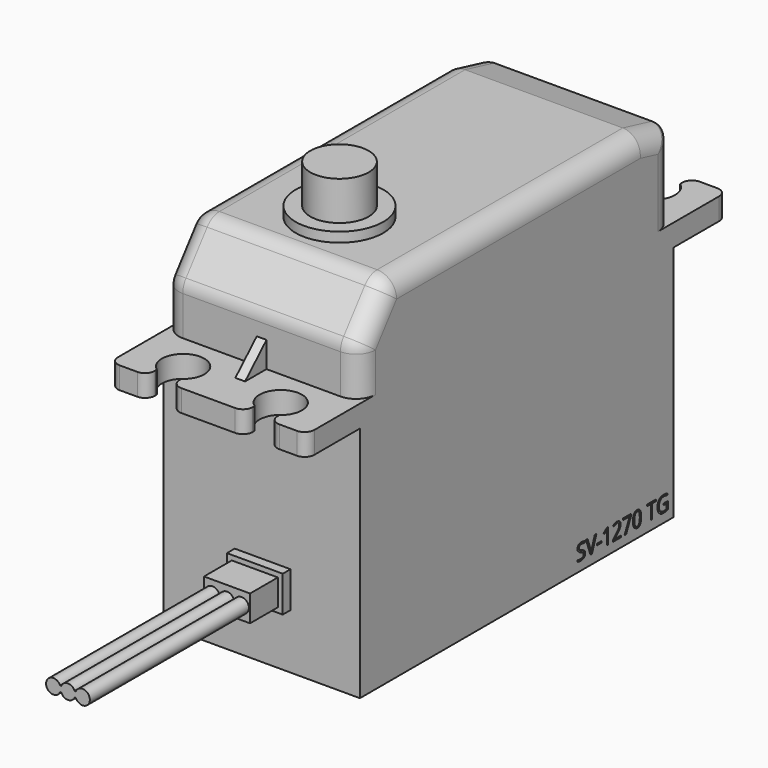
from build123d import *

# Parameters (mm, degrees)
F0_W          = 40.3
F0_H          = 24.4
F1_DEPTH      = 10.1
F2_DEPTH      = 0.5
F3_W          = 20.2
F3_H          = 27.65
F3_R          = 4.5
F3_H_2        = 5
F3_H_3        = 3
F4_DEPTH      = 1
F3_R_2        = 3
F5_DEPTH      = 4
F7_DEPTH      = 25
F8_R          = 2
F9_W          = 5.7326205064
F9_H          = 3.7
F9_W_2        = 4.7326205064
F9_H_2        = 2.7
F10_DEPTH     = 1
F11_DEPTH     = 4.57
F12_DEPTH     = 25
F13_TEXT_SIZE = 2.2495992416
F14_DEPTH     = 0.1
F15_R         = 0.5


# Not quite as in the source:
# - Text() gives the source's letters only with a copy of the font that has no kerning and outlines rounded to 1/6400 em; it was checked with that copy


with BuildPart() as f1:
    # F0 (on Right) → F1 (new body, symmetric)
    with BuildSketch(Plane.YZ):
        with Locations((0, -6.4)):
            Rectangle(F0_W, F0_H)
        Polygon((20.15, 8.05), (-20.15, 8.05), (-22.9002591223, 8.05), (-27, 8.05), (-27, 5.8), (-20.15, 5.8), (20.15, 5.8), (27.0000007004, 5.8), (27.0000007004, 8.05), (22.9000007004, 8.05), align=None)
        Polygon((12, 18.6), (-15.65, 18.6), (-20.15, 12.7771655098), (-20.15, 10.6946583837), (-20.15, 8.05), (20.15, 8.05), (20.15, 10.6946583837), (20.15, 16.6118297357), align=None)
    extrude(amount=F1_DEPTH, both=True)

    # F0 (on Right) → F2 (join, symmetric)
    with BuildSketch(Plane.YZ):
        Polygon((-20.15, 8.05), (-20.15, 10.6946583837), (-22.9002591223, 8.05), align=None)
        Polygon((22.9000007004, 8.05), (20.15, 10.6946583837), (20.15, 8.05), align=None)
    extrude(amount=F2_DEPTH, both=True)

    # F3 (on face) → F4 (cut)
    with BuildSketch(Plane.XY.offset(18.6)):
        with Locations((0, -1.825)):
            Rectangle(F3_W, F3_H)
        with Locations((0, -10.15)):
            Circle(F3_R, mode=Mode.SUBTRACT)
        with Locations((0, 14.5)):
            Rectangle(F3_W, F3_H_2)
        with Locations((0, -17.15)):
            Rectangle(F3_W, F3_H_3)
    extrude(amount=-F4_DEPTH, mode=Mode.SUBTRACT)

    # F3 (on face) → F5 (join)
    with BuildSketch(Plane.XY.offset(18.6)):
        with Locations((0, -10.15)):
            Circle(F3_R_2)
    extrude(amount=F5_DEPTH)

    # F6 (on Top) → F7 (cut)
    with BuildSketch(Plane.XY):
        with BuildLine():
            Line((0, -27), (0, -27.5084525347))
            Line((0, -27.5084525347), (10.378325358, -27.5084525347))
            Line((10.378325358, -27.5084525347), (10.378325358, -26))
            Line((10.378325358, -26), (10.1, -26))
            ThreePointArc((10.1, -26), (9.8071067812, -26.7071067812), (9.1, -27))
            Line((9.1, -27), (7.3, -27))
            ThreePointArc((7.3, -27), (6.5928932188, -26.7071067812), (6.3, -26))
            Line((6.3, -26), (6.3, -25.7791513451))
            ThreePointArc((6.3, -25.7791513451), (6.310365142, -25.734816345), (6.3393118446, -25.6996721164))
            ThreePointArc((6.3393118446, -25.6996721164), (4.9961864321, -21.7871178127), (3.7255205843, -25.7238011065))
            ThreePointArc((3.7255205843, -25.7238011065), (3.7555318396, -25.7592266373), (3.766310058, -25.8043871697))
            Line((3.766310058, -25.8043871697), (3.766310058, -26))
            ThreePointArc((3.766310058, -26), (3.4734168392, -26.7071067812), (2.766310058, -27))
            Line((2.766310058, -27), (0, -27))
        make_face()
        with BuildLine():
            Line((-10.378325358, -27.5084525347), (0, -27.5084525347))
            Line((0, -27.5084525347), (0, -27))
            Line((0, -27), (-2.766310058, -27))
            ThreePointArc((-2.766310058, -27), (-3.4734168392, -26.7071067812), (-3.766310058, -26))
            Line((-3.766310058, -26), (-3.766310058, -25.8043871697))
            ThreePointArc((-3.766310058, -25.8043871697), (-3.7555318396, -25.7592266373), (-3.7255205843, -25.7238011065))
            ThreePointArc((-3.7255205843, -25.7238011065), (-4.9961864321, -21.7871178127), (-6.3393118446, -25.6996721164))
            ThreePointArc((-6.3393118446, -25.6996721164), (-6.310365142, -25.734816345), (-6.3, -25.7791513451))
            Line((-6.3, -25.7791513451), (-6.3, -26))
            ThreePointArc((-6.3, -26), (-6.5928932188, -26.7071067812), (-7.3, -27))
            Line((-7.3, -27), (-9.1, -27))
            ThreePointArc((-9.1, -27), (-9.8071067812, -26.7071067812), (-10.1, -26))
            Line((-10.1, -26), (-10.378325358, -26))
            Line((-10.378325358, -26), (-10.378325358, -27.5084525347))
        make_face()
        with BuildLine():
            Line((10.378325358, 27.5084525347), (0, 27.5084525347))
            Line((0, 27.5084525347), (0, 27))
            Line((0, 27), (2.766310058, 27))
            ThreePointArc((2.766310058, 27), (3.4734168392, 26.7071067812), (3.766310058, 26))
            Line((3.766310058, 26), (3.766310058, 25.8043871697))
            ThreePointArc((3.766310058, 25.8043871697), (3.7555318396, 25.7592266373), (3.7255205843, 25.7238011065))
            ThreePointArc((3.7255205843, 25.7238011065), (4.9961864321, 21.7871178127), (6.3393118446, 25.6996721164))
            ThreePointArc((6.3393118446, 25.6996721164), (6.310365142, 25.734816345), (6.3, 25.7791513451))
            Line((6.3, 25.7791513451), (6.3, 26))
            ThreePointArc((6.3, 26), (6.5928932188, 26.7071067812), (7.3, 27))
            Line((7.3, 27), (9.1, 27))
            ThreePointArc((9.1, 27), (9.8071067812, 26.7071067812), (10.1, 26))
            Line((10.1, 26), (10.378325358, 26))
            Line((10.378325358, 26), (10.378325358, 27.5084525347))
        make_face()
        with BuildLine():
            Line((0, 27), (0, 27.5084525347))
            Line((0, 27.5084525347), (-10.378325358, 27.5084525347))
            Line((-10.378325358, 27.5084525347), (-10.378325358, 26))
            Line((-10.378325358, 26), (-10.1, 26))
            ThreePointArc((-10.1, 26), (-9.8071067812, 26.7071067812), (-9.1, 27))
            Line((-9.1, 27), (-7.3, 27))
            ThreePointArc((-7.3, 27), (-6.5928932188, 26.7071067812), (-6.3, 26))
            Line((-6.3, 26), (-6.3, 25.7791513451))
            ThreePointArc((-6.3, 25.7791513451), (-6.310365142, 25.734816345), (-6.3393118446, 25.6996721164))
            ThreePointArc((-6.3393118446, 25.6996721164), (-4.9961864321, 21.7871178127), (-3.7255205843, 25.7238011065))
            ThreePointArc((-3.7255205843, 25.7238011065), (-3.7555318396, 25.7592266373), (-3.766310058, 25.8043871697))
            Line((-3.766310058, 25.8043871697), (-3.766310058, 26))
            ThreePointArc((-3.766310058, 26), (-3.4734168392, 26.7071067812), (-2.766310058, 27))
            Line((-2.766310058, 27), (0, 27))
        make_face()
    extrude(amount=F7_DEPTH, mode=Mode.SUBTRACT)

    # F8
    f8_edges = [f1.edges().sort_by_distance(p)[0] for p in [
        (-10.1, 20.15, 12.330915),
        (-10.1, 18.124623, 17.105915),
        (-10.1, -0.161786, 17.6),
        (-10.1, -18.28641, 15.188583),
        (-10.1, -20.15, 10.413583),
        (10.1, 20.15, 12.330915),
        (10.1, 18.124623, 17.105915),
        (10.1, -0.161786, 17.6),
        (0, -20.15, 12.777166),
        (0, -16.422819, 17.6),
        (10.1, -20.15, 10.413583),
        (10.1, -18.28641, 15.188583),
    ]]
    fillet(f8_edges, radius=F8_R)

    # F9 (on face) → F10 (join)
    with BuildSketch(Plane.XZ.offset(20.15)):
        with Locations((0.1000001952, -11.1)):
            Rectangle(F9_W, F9_H)
        with Locations((0.1000001952, -11.1)):
            Rectangle(F9_W_2, F9_H_2, mode=Mode.SUBTRACT)
    extrude(amount=F10_DEPTH)

    # F9 (on face) → F11 (join)
    with BuildSketch(Plane.XZ.offset(20.15)):
        with Locations((0.1000001952, -11.1)):
            Rectangle(F9_W_2, F9_H_2)
        with BuildLine():
            ThreePointArc((0.7873865494, -11.4), (0.1000001952, -11.85), (-0.587386159, -11.4))
            Line((-0.587386159, -11.4), (-0.7126134506, -11.4))
            ThreePointArc((-0.7126134506, -11.4), (-2.1499998048, -11.0999998472), (-0.7126133283, -10.8000002801))
            Line((-0.7126133283, -10.8000002801), (-0.5873862813, -10.8000002801))
            ThreePointArc((-0.5873862813, -10.8000002801), (0.1000001952, -10.35), (0.7873866717, -10.8000002801))
            Line((0.7873866717, -10.8000002801), (0.9126137187, -10.8000002801))
            ThreePointArc((0.9126137187, -10.8000002801), (2.3500001952, -11.0999998472), (0.912613841, -11.4))
            Line((0.912613841, -11.4), (0.7873865494, -11.4))
        make_face(mode=Mode.SUBTRACT)
    extrude(amount=F11_DEPTH)

    # F9 (on face) → F12 (join)
    with BuildSketch(Plane.XZ.offset(20.15)):
        with BuildLine():
            Line((-0.7126134506, -11.4), (-0.587386159, -11.4))
            ThreePointArc((-0.587386159, -11.4), (0.1000001952, -11.85), (0.7873865494, -11.4))
            Line((0.7873865494, -11.4), (0.912613841, -11.4))
            ThreePointArc((0.912613841, -11.4), (2.3500001952, -11.0999998472), (0.9126137187, -10.8000002801))
            Line((0.9126137187, -10.8000002801), (0.7873866717, -10.8000002801))
            ThreePointArc((0.7873866717, -10.8000002801), (0.1000001952, -10.35), (-0.5873862813, -10.8000002801))
            Line((-0.5873862813, -10.8000002801), (-0.7126133283, -10.8000002801))
            ThreePointArc((-0.7126133283, -10.8000002801), (-2.1499998048, -11.0999998472), (-0.7126134506, -11.4))
        make_face()
    extrude(amount=F12_DEPTH)

    # F13 (on face) → F14 (cut)
    with BuildSketch(Plane.YZ.offset(10.1)):
        with Locations((7.6553690965, -17.6734838661)):
            Text('SV-1270 TG', F13_TEXT_SIZE, font='Open Sans', text_align=(TextAlign.LEFT, TextAlign.BOTTOM))
    extrude(amount=-F14_DEPTH, mode=Mode.SUBTRACT)

    # F15
    f15_edges = [f1.edges().sort_by_distance(p)[0] for p in [
        (0, 20.15, 16.61183),
    ]]
    fillet(f15_edges, radius=F15_R)


solid = f1.part
